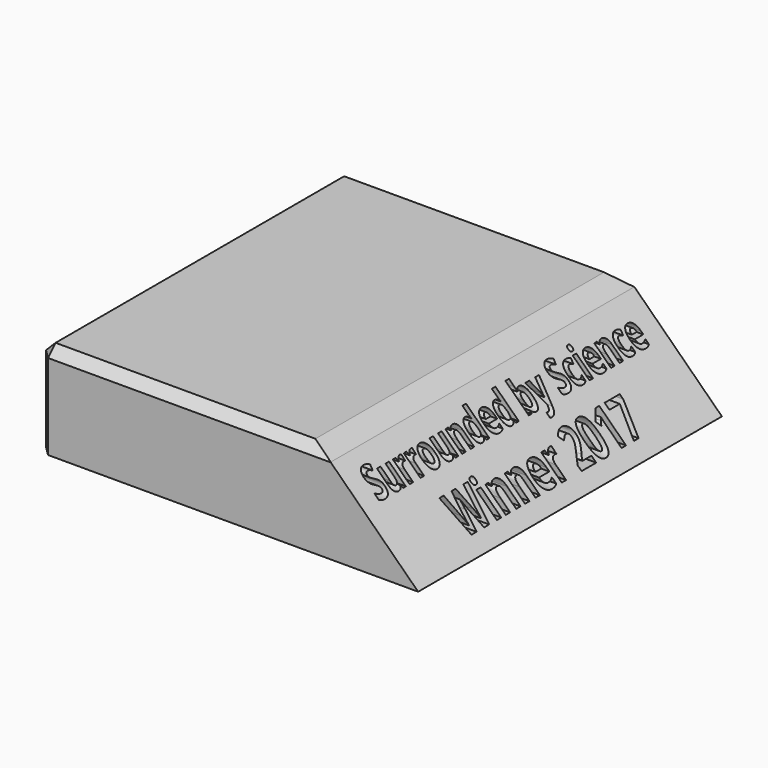
from build123d import *

# Parameters (mm, degrees)
F1_DEPTH       = 100
F2_TEXT_SIZE   = 7.9138272148
F2_TEXT_SIZE_2 = 9.6659702469
F3_DEPTH       = 47.3
F4_SIZE        = 2.5
F5_SIZE        = 3.5
F6_DEPTH       = 21


# Not quite as in the source:
# - Text() gives the source's letters only with a copy of the font that has no kerning and outlines rounded to 1/6400 em; it was checked with that copy


with BuildPart() as f1:
    # F0 (on Front) → F1 (new body)
    with BuildSketch(Plane.XZ):
        Polygon((50, -12.5), (24.4334433228, 12.5), (-50, 12.5), (-50, -12.5), align=None)
    extrude(amount=F1_DEPTH)

    # F2 (on Right) → F3 (cut)
    with BuildSketch(Plane.YZ):
        with Locations((-95, 1.5819507025)):
            Text('Surrounded by Science', F2_TEXT_SIZE, font='Open Sans', font_style=FontStyle.BOLD, text_align=(TextAlign.LEFT, TextAlign.BOTTOM))
        with Locations((-80, -9.2098470777)):
            Text('Winner 2017', F2_TEXT_SIZE_2, font='Open Sans', font_style=FontStyle.BOLD, text_align=(TextAlign.LEFT, TextAlign.BOTTOM))
    extrude(amount=F3_DEPTH, mode=Mode.SUBTRACT)

    # F4
    f4_edges = [f1.edges().sort_by_distance(p)[0] for p in [
        (-12.783278, -100, 12.5),
        (-50, -50, 12.5),
        (-12.783278, 0, 12.5),
        (-50, 0, 0),
        (-50, -100, 0),
    ]]
    chamfer(f4_edges, length=F4_SIZE)

    # F5
    f5_edges = [f1.edges().sort_by_distance(p)[0] for p in [
        (24.433443, -50, 12.5),
    ]]
    chamfer(f5_edges, length=F5_SIZE)

    # F2 (on Right) → F6 (join)
    with BuildSketch(Plane.YZ):
        with Locations((-95, 1.5819507025)):
            Text('Surrounded by Science', F2_TEXT_SIZE, font='Open Sans', font_style=FontStyle.BOLD, text_align=(TextAlign.LEFT, TextAlign.BOTTOM))
        with Locations((-80, -9.2098470777)):
            Text('Winner 2017', F2_TEXT_SIZE_2, font='Open Sans', font_style=FontStyle.BOLD, text_align=(TextAlign.LEFT, TextAlign.BOTTOM))
    extrude(amount=F6_DEPTH)


solid = f1.part
